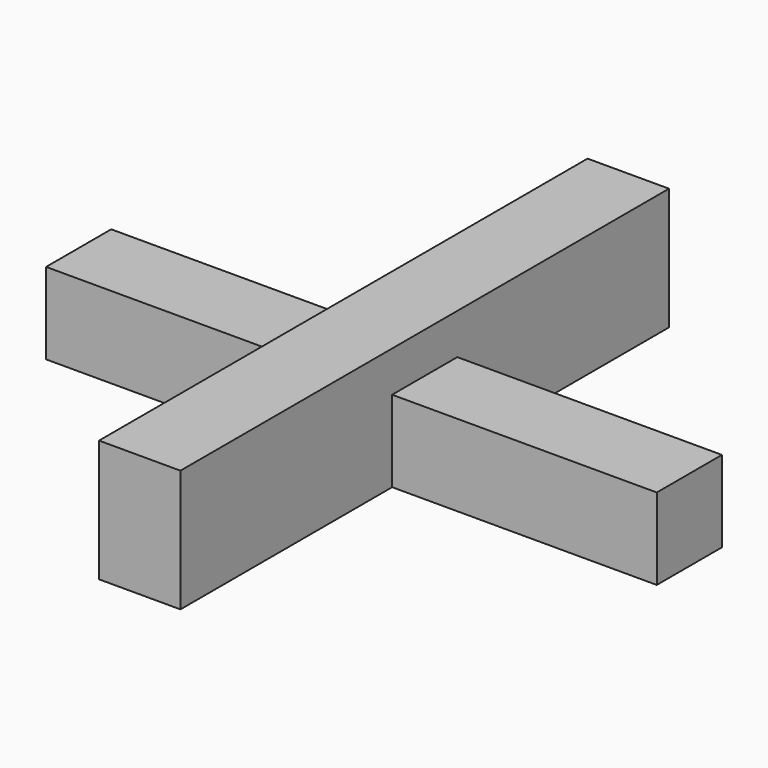
from build123d import *

# Parameters (mm, degrees)
F0_W     = 25.4
F0_H     = 82.55
F0_H_2   = 25.4
F1_DEPTH = 25.4
F0_W_2   = 82.55
F2_DEPTH = 12.7


with BuildPart() as f1:
    # F0 (on Top) → F1 (new body)
    with BuildSketch(Plane.XY):
        with Locations((0, 53.975)):
            Rectangle(F0_W, F0_H)
        Rectangle(F0_W, F0_H_2)
        with Locations((0, -53.975)):
            Rectangle(F0_W, F0_H)
    extrude(amount=F1_DEPTH)

    # F0 (on Top) → F2 (join, symmetric)
    with BuildSketch(Plane.XY):
        with Locations((0, 53.975)):
            Rectangle(F0_W, F0_H)
        Rectangle(F0_W, F0_H_2)
        with Locations((-53.975, 0)):
            Rectangle(F0_W_2, F0_H_2)
        with Locations((53.975, 0)):
            Rectangle(F0_W_2, F0_H_2)
        with Locations((0, -53.975)):
            Rectangle(F0_W, F0_H)
    extrude(amount=F2_DEPTH, both=True)


solid = f1.part
